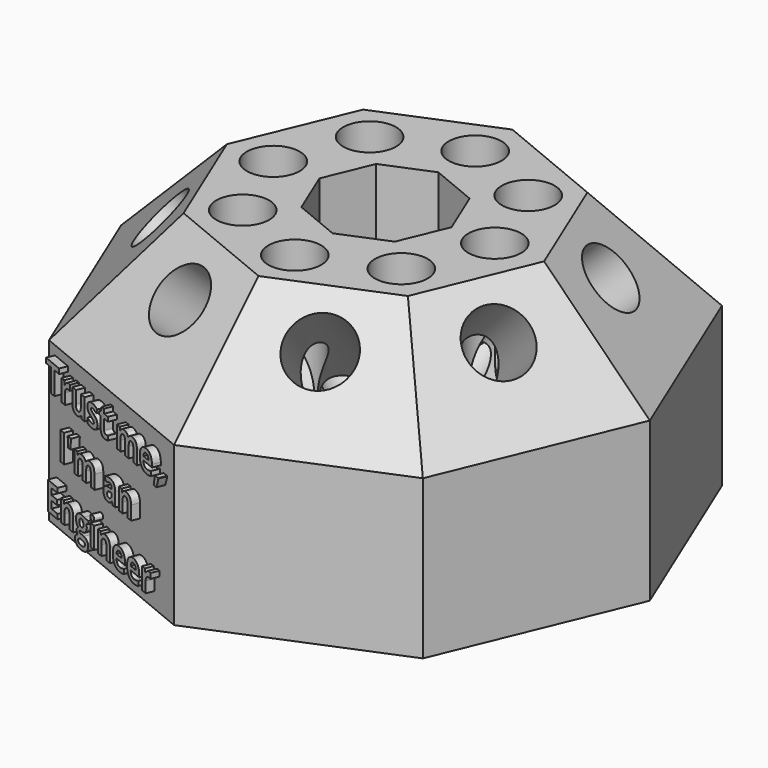
from build123d import *

# Parameters (mm, degrees)
F1_DEPTH      = 30
F5_R          = 6
F6_DEPTH      = 40
F7_R          = 6
F8_DEPTH      = 40
F9_R          = 6
F15_DEPTH     = 40
F10_R         = 6
F16_DEPTH     = 40
F11_R         = 6
F17_DEPTH     = 40
F12_R         = 6
F18_DEPTH     = 40
F13_R         = 6
F19_DEPTH     = 40
F14_R         = 6
F20_DEPTH     = 40
F21_R         = 5
F22_DEPTH     = 40
F23_DEPTH     = 20
F24_TEXT_SIZE = 7.3795875338
F25_DEPTH     = 1.5


# Not quite as in the source:
# - Text() gives the source's letters only with a copy of the font that has no kerning and outlines rounded to 1/6400 em; it was checked with that copy


with BuildPart() as f1:
    # F0 (on Top) → F1 (new body)
    with BuildSketch(Plane.XY):
        Polygon((-35.3553390593, -35.3553390593), (0, -50), (35.3553390593, -35.3553390593), (50, 0), (35.3553390593, 35.3553390593), (0, 50), (-35.3553390593, 35.3553390593), (-50, 0), align=None)
    extrude(amount=F1_DEPTH)

    # F1_face (on face) → F4 section 0
    with BuildSketch(Plane.XY.offset(30)):
        Polygon((-35.3553390593, -35.3553390593), (0, -50), (35.3553390593, -35.3553390593), (50, 0), (35.3553390593, 35.3553390593), (0, 50), (-35.3553390593, 35.3553390593), (-50, 0), align=None)
    # F3 (on offset) → F4 section 1
    with BuildSketch(Plane.XY.offset(50)):
        Polygon((-21.2132034356, -21.2132034356), (0, -30), (21.2132034356, -21.2132034356), (30, 0), (21.2132034356, 21.2132034356), (0, 30), (-21.2132034356, 21.2132034356), (-30, 0), align=None)
    loft()

    # F5 (on face) → F6 (cut)
    with BuildSketch(Plane(origin=(-36.8396570576, -15.2594855864, 36.8396570576), x_dir=(0.7345095553, -0.2596883437, 0.6269431213), z_dir=(-0.6785983445, -0.2810846377, 0.6785983445))):
        with Locations((6.5777291469, 4.0150180798)):
            Circle(F5_R)
    extrude(amount=-F6_DEPTH, mode=Mode.SUBTRACT)

    # F7 (on face) → F8 (cut)
    with BuildSketch(Plane(origin=(-15.2594855864, -36.8396570576, 36.8396570576), x_dir=(0.9596829823, -0.1987568534, 0.1987568534), z_dir=(-0.2810846377, -0.6785983445, 0.6785983445))):
        with Locations((2.08530679, 7.4187860532)):
            Circle(F7_R)
    extrude(amount=-F8_DEPTH, mode=Mode.SUBTRACT)

    # F9 (on face) → F15 (cut)
    with BuildSketch(Plane(origin=(15.2594855864, -36.8396570576, 36.8396570576), x_dir=(0.9596829823, 0.1987568534, -0.1987568534), z_dir=(0.2810846377, -0.6785983445, 0.6785983445))):
        with Locations((-2.08530679, 7.4187860532)):
            Circle(F9_R)
    extrude(amount=-F15_DEPTH, mode=Mode.SUBTRACT)

    # F10 (on face) → F16 (cut)
    with BuildSketch(Plane(origin=(36.8396570576, -15.2594855864, 36.8396570576), x_dir=(0.1987568534, 0.9596829823, 0.1987568534), z_dir=(0.6785983445, -0.2810846377, 0.6785983445))):
        with Locations((2.08530679, 7.4187860532)):
            Circle(F10_R)
    extrude(amount=-F16_DEPTH, mode=Mode.SUBTRACT)

    # F11 (on face) → F17 (cut)
    with BuildSketch(Plane(origin=(36.8396570576, 15.2594855864, 36.8396570576), x_dir=(-0.1987568534, 0.9596829823, -0.1987568534), z_dir=(0.6785983445, 0.2810846377, 0.6785983445))):
        with Locations((-2.08530679, 7.4187860532)):
            Circle(F11_R)
    extrude(amount=-F17_DEPTH, mode=Mode.SUBTRACT)

    # F12 (on face) → F18 (cut)
    with BuildSketch(Plane(origin=(15.2594855864, 36.8396570576, 36.8396570576), x_dir=(-0.9596829823, 0.1987568534, 0.1987568534), z_dir=(0.2810846377, 0.6785983445, 0.6785983445))):
        with Locations((2.08530679, 7.4187860532)):
            Circle(F12_R)
    extrude(amount=-F18_DEPTH, mode=Mode.SUBTRACT)

    # F13 (on face) → F19 (cut)
    with BuildSketch(Plane(origin=(-15.2594855864, 36.8396570576, 36.8396570576), x_dir=(-0.9596829823, -0.1987568534, -0.1987568534), z_dir=(-0.2810846377, 0.6785983445, 0.6785983445))):
        with Locations((-2.08530679, 7.4187860532)):
            Circle(F13_R)
    extrude(amount=-F19_DEPTH, mode=Mode.SUBTRACT)

    # F14 (on face) → F20 (cut)
    with BuildSketch(Plane(origin=(-36.8396570576, 15.2594855864, 36.8396570576), x_dir=(-0.1987568534, -0.9596829823, 0.1987568534), z_dir=(-0.6785983445, 0.2810846377, 0.6785983445))):
        with Locations((2.08530679, 7.4187860532)):
            Circle(F14_R)
    extrude(amount=-F20_DEPTH, mode=Mode.SUBTRACT)

    # F21 (on face) → F22 (cut)
    with BuildSketch(Plane.XY.offset(50)):
        with Locations((0, 21.2132034356)):
            Circle(F21_R)
        with Locations((-15, 15)):
            Circle(F21_R)
        with Locations((-21.2132034356, 0)):
            Circle(F21_R)
        with Locations((-15, -15)):
            Circle(F21_R)
        with Locations((0, -21.4324984606)):
            Circle(F21_R)
        with Locations((15, -15)):
            Circle(F21_R)
        with Locations((20.6860724459, 0)):
            Circle(F21_R)
        with Locations((15, 15)):
            Circle(F21_R)
    extrude(amount=-F22_DEPTH, mode=Mode.SUBTRACT)

    # F21 (on face) → F23 (cut)
    with BuildSketch(Plane.XY.offset(50)):
        Polygon((-8.8388347648, 8.8388347648), (-12.5, 0), (-8.8388347648, -8.8388347648), (0, -12.5), (8.8388347648, -8.8388347648), (12.5, 0), (8.8388347648, 8.8388347648), (0, 12.5), align=None)
    extrude(amount=-F23_DEPTH, mode=Mode.SUBTRACT)

    # F24 (on face) → F25 (join)
    with BuildSketch(Plane(origin=(-17.6776695297, -42.6776695297, 0), x_dir=(0.9238795325, -0.3826834324, 0), z_dir=(-0.3826834324, -0.9238795325, 0))):
        with Locations((-17.4578177478, 23.0379570618)):
            Text('Trust me,', F24_TEXT_SIZE, font='Open Sans', font_style=FontStyle.BOLD, text_align=(TextAlign.LEFT, TextAlign.BOTTOM))
        with Locations((-13.6227383514, 13.0017180159)):
            Text("I'm an", F24_TEXT_SIZE, font='Open Sans', font_style=FontStyle.BOLD, text_align=(TextAlign.LEFT, TextAlign.BOTTOM))
        with Locations((-17.4578177478, 2.96547897)):
            Text('Engineer', F24_TEXT_SIZE, font='Open Sans', font_style=FontStyle.BOLD, text_align=(TextAlign.LEFT, TextAlign.BOTTOM))
    extrude(amount=F25_DEPTH)


solid = f1.part
